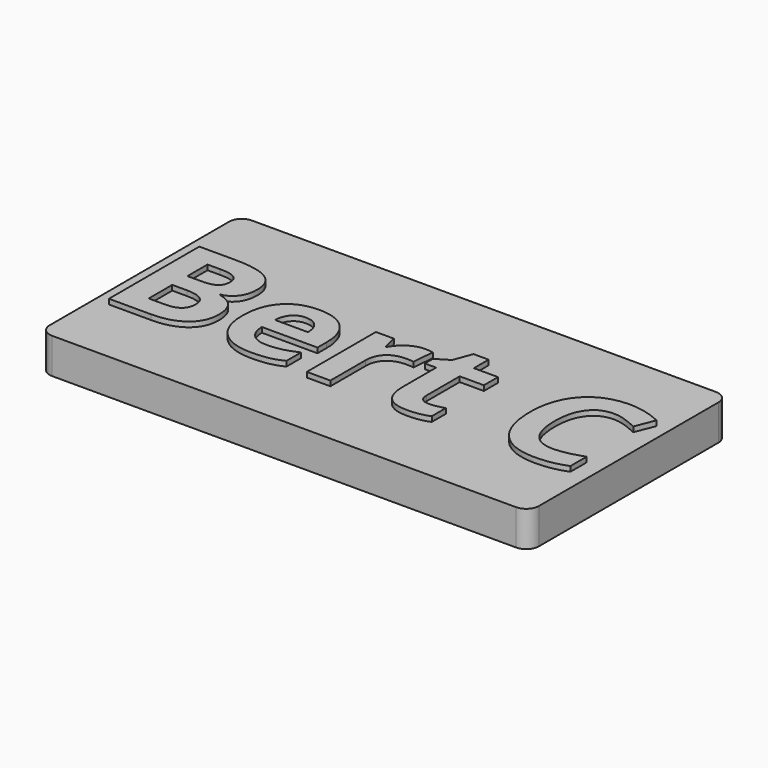
from build123d import *

# Parameters (mm, degrees)
F0_W         = 38.6
F0_H         = 19.7
F0_TEXT_SIZE = 12.4806804626
F1_DEPTH     = 2.8
F2_DEPTH     = 3.2
F3_R         = 1


# Not quite as in the source:
# - Text() gives the source's letters only with a copy of the font that has no kerning and outlines rounded to 1/6400 em; it was checked with that copy


with BuildPart() as f1:
    # F0 (on Top) → F1 (new body)
    with BuildSketch(Plane.XY):
        with Locations((-4.5407602289, 9.85)):
            Rectangle(F0_W, F0_H)
        with BuildLine():
            add(Edge.make_bspline(
                [(-10.0437579988, 5.4416370639), (-10.5975881943, 5.3226805782), (-11.3971317864, 5.3226805782)],
                knots=[0, 0, 0, 1, 1, 1], degree=2))
            add(Edge.make_bspline(
                [(-11.3971317864, 5.3226805782), (-13.0410714161, 5.3226805782), (-13.9673719192, 6.2314301244)],
                knots=[0, 0, 0, 1, 1, 1], degree=2))
            add(Edge.make_bspline(
                [(-13.9673719192, 6.2314301244), (-14.8936724223, 7.1401796706), (-14.8936724223, 8.8036203635)],
                knots=[0, 0, 0, 1, 1, 1], degree=2))
            add(Edge.make_bspline(
                [(-14.8936724223, 8.8036203635), (-14.8936724223, 10.5158137144), (-14.0375757468, 11.450889696)],
                knots=[0, 0, 0, 1, 1, 1], degree=2))
            add(Edge.make_bspline(
                [(-14.0375757468, 11.450889696), (-13.1814790713, 12.3859656775), (-11.6701466716, 12.3859656775)],
                knots=[0, 0, 0, 1, 1, 1], degree=2))
            add(Edge.make_bspline(
                [(-11.6701466716, 12.3859656775), (-10.2270679931, 12.3859656775), (-9.4226491351, 11.5639958627)],
                knots=[0, 0, 0, 1, 1, 1], degree=2))
            add(Edge.make_bspline(
                [(-9.4226491351, 11.5639958627), (-8.6182302772, 10.7420260478), (-8.6182302772, 9.291146944)],
                knots=[0, 0, 0, 1, 1, 1], degree=2))
            Line((-8.6182302772, 9.291146944), (-8.6182302772, 8.3882477168))
            Line((-8.6182302772, 8.3882477168), (-13.0118198213, 8.3882477168))
            add(Edge.make_bspline(
                [(-13.0118198213, 8.3882477168), (-12.9806181201, 7.59650455), (-12.5418441976, 7.1518803085)],
                knots=[0, 0, 0, 1, 1, 1], degree=2))
            add(Edge.make_bspline(
                [(-12.5418441976, 7.1518803085), (-12.1030702751, 6.707256067), (-11.3113271083, 6.707256067)],
                knots=[0, 0, 0, 1, 1, 1], degree=2))
            add(Edge.make_bspline(
                [(-11.3113271083, 6.707256067), (-10.6950935104, 6.707256067), (-10.1471136338, 6.8349880311)],
                knots=[0, 0, 0, 1, 1, 1], degree=2))
            add(Edge.make_bspline(
                [(-10.1471136338, 6.8349880311), (-9.5991337573, 6.9627199952), (-9.0024012227, 7.2435353056)],
                knots=[0, 0, 0, 1, 1, 1], degree=2))
            Line((-9.0024012227, 7.2435353056), (-9.0024012227, 5.8043568398))
            add(Edge.make_bspline(
                [(-9.0024012227, 5.8043568398), (-9.4899278032, 5.5605935495), (-10.0437579988, 5.4416370639)],
                knots=[0, 0, 0, 1, 1, 1], degree=2))
        make_face(mode=Mode.SUBTRACT)
        with BuildLine():
            add(Edge.make_bspline(
                [(-4.4771795018, 12.0359215927), (-3.9379751037, 12.3859656775), (-3.3041905489, 12.3859656775)],
                knots=[0, 0, 0, 1, 1, 1], degree=2))
            add(Edge.make_bspline(
                [(-3.3041905489, 12.3859656775), (-2.9258699224, 12.3859656775), (-2.6762563132, 12.3313627005)],
                knots=[0, 0, 0, 1, 1, 1], degree=2))
            Line((-2.6762563132, 12.3313627005), (-2.8166639684, 10.5899177547))
            add(Edge.make_bspline(
                [(-2.8166639684, 10.5899177547), (-3.0428763018, 10.6503710507), (-3.3646438449, 10.6503710507)],
                knots=[0, 0, 0, 1, 1, 1], degree=2))
            add(Edge.make_bspline(
                [(-3.3646438449, 10.6503710507), (-4.2538923279, 10.6503710507), (-4.7511694401, 10.1930711181)],
                knots=[0, 0, 0, 1, 1, 1], degree=2))
            add(Edge.make_bspline(
                [(-4.7511694401, 10.1930711181), (-5.2484465523, 9.7357711855), (-5.2484465523, 8.9128263175)],
                knots=[0, 0, 0, 1, 1, 1], degree=2))
            Line((-5.2484465523, 8.9128263175), (-5.2484465523, 5.4455372765))
            Line((-5.2484465523, 5.4455372765), (-7.1068978774, 5.4455372765))
            Line((-7.1068978774, 5.4455372765), (-7.1068978774, 12.2592087666))
            Line((-7.1068978774, 12.2592087666), (-5.6989211127, 12.2592087666))
            Line((-5.6989211127, 12.2592087666), (-5.4239561213, 11.1125462491))
            Line((-5.4239561213, 11.1125462491), (-5.3342512304, 11.1125462491))
            add(Edge.make_bspline(
                [(-5.3342512304, 11.1125462491), (-5.0163838999, 11.6858775078), (-4.4771795018, 12.0359215927)],
                knots=[0, 0, 0, 1, 1, 1], degree=2))
        make_face(mode=Mode.SUBTRACT)
        with BuildLine():
            add(Edge.make_bspline(
                [(0.8417354922, 6.9939216964), (1.064047613, 6.8047613831), (1.4306676016, 6.8047613831)],
                knots=[0, 0, 0, 1, 1, 1], degree=2))
            add(Edge.make_bspline(
                [(1.4306676016, 6.8047613831), (1.9181941821, 6.8047613831), (2.6007313949, 7.0173229723)],
                knots=[0, 0, 0, 1, 1, 1], degree=2))
            Line((2.6007313949, 7.0173229723), (2.6007313949, 5.6346975898))
            add(Edge.make_bspline(
                [(2.6007313949, 5.6346975898), (1.9064935442, 5.3226805782), (0.8943883629, 5.3226805782)],
                knots=[0, 0, 0, 1, 1, 1], degree=2))
            add(Edge.make_bspline(
                [(0.8943883629, 5.3226805782), (-0.2210724534, 5.3226805782), (-0.7300502035, 5.8872363585)],
                knots=[0, 0, 0, 1, 1, 1], degree=2))
            add(Edge.make_bspline(
                [(-0.7300502035, 5.8872363585), (-1.2390279536, 6.4517921388), (-1.2390279536, 7.5789535931)],
                knots=[0, 0, 0, 1, 1, 1], degree=2))
            Line((-1.2390279536, 7.5789535931), (-1.2390279536, 10.8629326398))
            Line((-1.2390279536, 10.8629326398), (-2.1282764366, 10.8629326398))
            Line((-2.1282764366, 10.8629326398), (-2.1282764366, 11.6488254877))
            Line((-2.1282764366, 11.6488254877), (-1.1044706174, 12.2709094045))
            Line((-1.1044706174, 12.2709094045), (-0.5681913788, 13.7100878703))
            Line((-0.5681913788, 13.7100878703), (0.6194233715, 13.7100878703))
            Line((0.6194233715, 13.7100878703), (0.6194233715, 12.2592087666))
            Line((0.6194233715, 12.2592087666), (2.5266273547, 12.2592087666))
            Line((2.5266273547, 12.2592087666), (2.5266273547, 10.8629326398))
            Line((2.5266273547, 10.8629326398), (0.6194233715, 10.8629326398))
            Line((0.6194233715, 10.8629326398), (0.6194233715, 7.5789535931))
            add(Edge.make_bspline(
                [(0.6194233715, 7.5789535931), (0.6194233715, 7.1830820097), (0.8417354922, 6.9939216964)],
                knots=[0, 0, 0, 1, 1, 1], degree=2))
        make_face(mode=Mode.SUBTRACT)
        with BuildLine():
            Line((-22.7194490936, 5.4455372765), (-22.7194490936, 14.355573063))
            Line((-22.7194490936, 14.355573063), (-19.9463979033, 14.355573063))
            add(Edge.make_bspline(
                [(-19.9463979033, 14.355573063), (-18.0508945581, 14.355573063), (-17.1947978826, 13.8163686649)],
                knots=[0, 0, 0, 1, 1, 1], degree=2))
            add(Edge.make_bspline(
                [(-17.1947978826, 13.8163686649), (-16.3387012071, 13.2771642668), (-16.3387012071, 12.1012501545)],
                knots=[0, 0, 0, 1, 1, 1], degree=2))
            add(Edge.make_bspline(
                [(-16.3387012071, 12.1012501545), (-16.3387012071, 11.3017065623), (-16.713121621, 10.7898036527)],
                knots=[0, 0, 0, 1, 1, 1], degree=2))
            add(Edge.make_bspline(
                [(-16.713121621, 10.7898036527), (-17.0875420349, 10.2779007431), (-17.7096259517, 10.174545108)],
                knots=[0, 0, 0, 1, 1, 1], degree=2))
            Line((-17.7096259517, 10.174545108), (-17.7096259517, 10.114091812))
            add(Edge.make_bspline(
                [(-17.7096259517, 10.114091812), (-16.8632798078, 9.9249314988), (-16.4878843408, 9.4071782702)],
                knots=[0, 0, 0, 1, 1, 1], degree=2))
            add(Edge.make_bspline(
                [(-16.4878843408, 9.4071782702), (-16.1124888737, 8.8894250417), (-16.1124888737, 8.0294281535)],
                knots=[0, 0, 0, 1, 1, 1], degree=2))
            add(Edge.make_bspline(
                [(-16.1124888737, 8.0294281535), (-16.1124888737, 6.8106117021), (-16.9939369314, 6.1280744893)],
                knots=[0, 0, 0, 1, 1, 1], degree=2))
            add(Edge.make_bspline(
                [(-16.9939369314, 6.1280744893), (-17.8753849891, 5.4455372765), (-19.3867173888, 5.4455372765)],
                knots=[0, 0, 0, 1, 1, 1], degree=2))
            Line((-19.3867173888, 5.4455372765), (-22.7194490936, 5.4455372765))
        make_face(mode=Mode.SUBTRACT)
        with BuildLine():
            add(Edge.make_bspline(
                [(12.1445517362, 12.734059656), (11.6394741987, 12.9105442782), (11.1519476182, 12.9105442782)],
                knots=[0, 0, 0, 1, 1, 1], degree=2))
            add(Edge.make_bspline(
                [(11.1519476182, 12.9105442782), (10.0852394599, 12.9105442782), (9.5002075632, 12.1090505797)],
                knots=[0, 0, 0, 1, 1, 1], degree=2))
            add(Edge.make_bspline(
                [(9.5002075632, 12.1090505797), (8.9151756665, 11.3075568813), (8.9151756665, 9.8761788407)],
                knots=[0, 0, 0, 1, 1, 1], degree=2))
            add(Edge.make_bspline(
                [(8.9151756665, 9.8761788407), (8.9151756665, 6.8964163803), (11.1519476182, 6.8964163803)],
                knots=[0, 0, 0, 1, 1, 1], degree=2))
            add(Edge.make_bspline(
                [(11.1519476182, 6.8964163803), (12.0899487592, 6.8964163803), (13.4238214836, 7.3644418976)],
                knots=[0, 0, 0, 1, 1, 1], degree=2))
            Line((13.4238214836, 7.3644418976), (13.4238214836, 5.7809555639))
            add(Edge.make_bspline(
                [(13.4238214836, 5.7809555639), (12.3278617305, 5.3226805782), (10.9744879428, 5.3226805782)],
                knots=[0, 0, 0, 1, 1, 1], degree=2))
            add(Edge.make_bspline(
                [(10.9744879428, 5.3226805782), (9.0302319395, 5.3226805782), (8.0005758013, 6.5024949032)],
                knots=[0, 0, 0, 1, 1, 1], degree=2))
            add(Edge.make_bspline(
                [(8.0005758013, 6.5024949032), (6.9709196632, 7.6823092282), (6.9709196632, 9.8878794787)],
                knots=[0, 0, 0, 1, 1, 1], degree=2))
            add(Edge.make_bspline(
                [(6.9709196632, 9.8878794787), (6.9709196632, 11.2783052865), (7.4769722538, 12.3235622752)],
                knots=[0, 0, 0, 1, 1, 1], degree=2))
            add(Edge.make_bspline(
                [(7.4769722538, 12.3235622752), (7.9830248444, 13.3688192639), (8.9307765171, 13.925574619)],
                knots=[0, 0, 0, 1, 1, 1], degree=2))
            add(Edge.make_bspline(
                [(8.9307765171, 13.925574619), (9.8785281897, 14.482329974), (11.1519476182, 14.482329974)],
                knots=[0, 0, 0, 1, 1, 1], degree=2))
            add(Edge.make_bspline(
                [(11.1519476182, 14.482329974), (12.4487683225, 14.482329974), (13.7592397711, 13.8563458445)],
                knots=[0, 0, 0, 1, 1, 1], degree=2))
            Line((13.7592397711, 13.8563458445), (13.1508065985, 12.3196620626))
            add(Edge.make_bspline(
                [(13.1508065985, 12.3196620626), (12.6496292737, 12.5575750339), (12.1445517362, 12.734059656)],
                knots=[0, 0, 0, 1, 1, 1], degree=2))
        make_face(mode=Mode.SUBTRACT)
        with BuildLine():
            Line((-20.8297960673, 12.8071886431), (-20.8297960673, 10.8258806197))
            Line((-20.8297960673, 10.8258806197), (-19.7338363142, 10.8258806197))
            add(Edge.make_bspline(
                [(-19.7338363142, 10.8258806197), (-18.9654944232, 10.8258806197), (-18.6213006573, 11.063793591)],
                knots=[0, 0, 0, 1, 1, 1], degree=2))
            add(Edge.make_bspline(
                [(-18.6213006573, 11.063793591), (-18.2771068915, 11.3017065623), (-18.2771068915, 11.8496864389)],
                knots=[0, 0, 0, 1, 1, 1], degree=2))
            add(Edge.make_bspline(
                [(-18.2771068915, 11.8496864389), (-18.2771068915, 12.3625644016), (-18.6515273053, 12.5848765224)],
                knots=[0, 0, 0, 1, 1, 1], degree=2))
            add(Edge.make_bspline(
                [(-18.6515273053, 12.5848765224), (-19.0259477192, 12.8071886431), (-19.8371919493, 12.8071886431)],
                knots=[0, 0, 0, 1, 1, 1], degree=2))
            Line((-19.8371919493, 12.8071886431), (-20.8297960673, 12.8071886431))
        make_face()
        with BuildLine():
            Line((-19.659732274, 9.3281989642), (-20.8297960673, 9.3281989642))
            Line((-20.8297960673, 9.3281989642), (-20.8297960673, 7.0056223343))
            Line((-20.8297960673, 7.0056223343), (-19.599278978, 7.0056223343))
            add(Edge.make_bspline(
                [(-19.599278978, 7.0056223343), (-18.8192364491, 7.0056223343), (-18.4477411947, 7.3039886016)],
                knots=[0, 0, 0, 1, 1, 1], degree=2))
            add(Edge.make_bspline(
                [(-18.4477411947, 7.3039886016), (-18.0762459403, 7.6023548689), (-18.0762459403, 8.2185884668)],
                knots=[0, 0, 0, 1, 1, 1], degree=2))
            add(Edge.make_bspline(
                [(-18.0762459403, 8.2185884668), (-18.0762459403, 9.3281989642), (-19.659732274, 9.3281989642)],
                knots=[0, 0, 0, 1, 1, 1], degree=2))
        make_face()
        with BuildLine():
            add(Edge.make_bspline(
                [(-10.7204448926, 10.6893731771), (-11.067563818, 11.063793591), (-11.6584460336, 11.063793591)],
                knots=[0, 0, 0, 1, 1, 1], degree=2))
            add(Edge.make_bspline(
                [(-11.6584460336, 11.063793591), (-12.2493282493, 11.063793591), (-12.5847465367, 10.6893731771)],
                knots=[0, 0, 0, 1, 1, 1], degree=2))
            add(Edge.make_bspline(
                [(-12.5847465367, 10.6893731771), (-12.9201648241, 10.3149527632), (-12.9689174822, 9.6265652315)],
                knots=[0, 0, 0, 1, 1, 1], degree=2))
            Line((-12.9689174822, 9.6265652315), (-10.359675223, 9.6265652315))
            add(Edge.make_bspline(
                [(-10.359675223, 9.6265652315), (-10.3733259672, 10.3149527632), (-10.7204448926, 10.6893731771)],
                knots=[0, 0, 0, 1, 1, 1], degree=2))
        make_face()
        with Locations((-23.8407602289, 5.4455372765)):
            Text('Bert C', F0_TEXT_SIZE, font='Open Sans', font_style=FontStyle.BOLD, text_align=(TextAlign.LEFT, TextAlign.BOTTOM))
    extrude(amount=F1_DEPTH)

    # F0 (on Top) → F2 (join)
    with BuildSketch(Plane.XY):
        with Locations((-23.8407602289, 5.4455372765)):
            Text('Bert C', F0_TEXT_SIZE, font='Open Sans', font_style=FontStyle.BOLD, text_align=(TextAlign.LEFT, TextAlign.BOTTOM))
    extrude(amount=F2_DEPTH)

    # F3
    f3_edges = [f1.edges().sort_by_distance(p)[0] for p in [
        (14.75924, 0, 1.4),
        (14.75924, 19.7, 1.4),
        (-23.84076, 0, 1.4),
        (-23.84076, 19.7, 1.4),
    ]]
    fillet(f3_edges, radius=F3_R)


solid = f1.part
